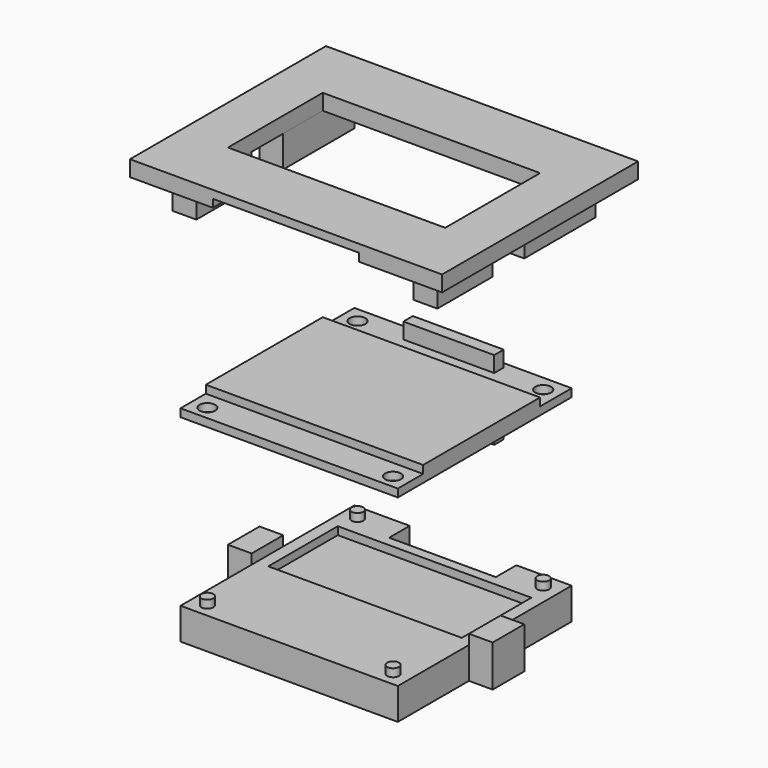
from build123d import *

# Parameters (mm, degrees)
F0_W          = 27.5
F0_H          = 27.5
F0_R          = 1
F1_DEPTH      = 1
F2_W          = 18.5
F2_H          = 1
F3_DEPTH      = 13.75
F3_DEPTH_BACK = 13.75
F4_W          = 11.5
F4_H          = 1.5
F5_DEPTH      = 2
F5_DEPTH_BACK = 8
F6_W          = 23.5
F6_H          = 10
F7_DEPTH      = 0.5
F9_W          = 39.5
F9_H          = 31
F9_W_2        = 27.5000000002
F9_H_2        = 3.5
F10_DEPTH     = 2
F11_W         = 27.5
F11_H         = 3.5
F11_H_2       = 4.5
F11_W_2       = 12.5
F11_H_3       = 2.5
F11_W_3       = 11.5
F11_H_4       = 1.5
F12_DEPTH     = 1
F13_W         = 3
F13_H         = 8.75
F14_DEPTH     = 4
F15_W         = 4.5
F15_H         = 3.5
F16_DEPTH     = 1
F18_W         = 33.5
F18_H         = 27.5
F19_DEPTH     = 4
F20_R         = 0.75
F21_DEPTH     = 1
F22_W         = 3
F22_H         = 5
F23_DEPTH     = 1.25
F24_W         = 3
F24_H         = 11.25
F24_W_2       = 13.5
F24_H_2       = 3.25
F25_DEPTH     = 4
F26_W         = 24.5
F26_H         = 11
F27_DEPTH     = 1


with BuildPart() as f1:
    # F0 (on Top) → F1 (new body)
    with BuildSketch(Plane.XY):
        Rectangle(F0_W, F0_H)
        with Locations((-11.75, -12)):
            Circle(F0_R, mode=Mode.SUBTRACT)
        with Locations((11.75, -12)):
            Circle(F0_R, mode=Mode.SUBTRACT)
        with Locations((-11.75, 11.75)):
            Circle(F0_R, mode=Mode.SUBTRACT)
        with Locations((11.75, 11.75)):
            Circle(F0_R, mode=Mode.SUBTRACT)
    extrude(amount=F1_DEPTH)

    # F2 (on Right) → F3 (join, two sides)
    with BuildSketch(Plane.YZ) as f3_sk:
        with Locations((-0.5, 1.5)):
            Rectangle(F2_W, F2_H)
    extrude(amount=F3_DEPTH)
    extrude(f3_sk.sketch, amount=-F3_DEPTH_BACK)

    # F4 (on face) → F5 (join, two sides)
    with BuildSketch(Plane.XY.offset(1)) as f5_sk:
        with Locations((0, 12.25)):
            Rectangle(F4_W, F4_H)
    extrude(amount=F5_DEPTH)
    extrude(f5_sk.sketch, amount=-F5_DEPTH_BACK)

    # F6 (on face) → F7 (join)
    with BuildSketch(Plane(origin=(0, 0, 0), x_dir=(1, 0, 0), z_dir=(0, 0, -1))):
        with Locations((0, -3.75)):
            Rectangle(F6_W, F6_H)
    extrude(amount=F7_DEPTH)


with BuildPart() as f10:
    # F9 (on offset) → F10 (new body)
    with BuildSketch(Plane.XY.offset(25)):
        with Locations((0, 1.25)):
            Rectangle(F9_W, F9_H)
        Polygon((-13.7499999998, 8.75), (13.7500000002, 8.75), (13.75, -6.25), (13.75, -9.75), (-13.7499999998, -9.75), (-13.75, -6.25), align=None, mode=Mode.SUBTRACT)
        with Locations((1e-10, -8)):
            Rectangle(F9_W_2, F9_H_2)
    extrude(amount=F10_DEPTH)

    # F11 (on face) → F12 (cut)
    with BuildSketch(Plane(origin=(0, 0, 25), x_dir=(1, 0, 0), z_dir=(0, 0, -1))):
        with Locations((0, 8)):
            Rectangle(F11_W, F11_H)
        with Locations((0, 12)):
            Rectangle(F11_W, F11_H_2)
        with Locations((0, -12.25)):
            Rectangle(F11_W_2, F11_H_3)
        with Locations((0, -12.25)):
            Rectangle(F11_W_3, F11_H_4, mode=Mode.SUBTRACT)
        with Locations((0, -12.25)):
            Rectangle(F11_W_3, F11_H_4)
    extrude(amount=-F12_DEPTH, mode=Mode.SUBTRACT)

    # F13 (on face) → F14 (join)
    with BuildSketch(Plane(origin=(0, 0, 25), x_dir=(1, 0, 0), z_dir=(0, 0, -1))):
        with Locations((-15.25, 6.875)):
            Rectangle(F13_W, F13_H)
        Polygon((16.75, -2.5), (13.75, -2.5), (13.75, -8.75), (13.75, -13.75), (16.75, -13.75), align=None)
        Polygon((-13.75, -8.75), (-13.75, -2.5), (-16.75, -2.5), (-16.75, -13.75), (-13.75, -13.75), align=None)
        with Locations((15.25, 6.875)):
            Rectangle(F13_W, F13_H)
    extrude(amount=F14_DEPTH)

    # F15 (on face) → F16 (join, through all)
    with BuildSketch(Plane(origin=(0, 0, 26), x_dir=(1, 0, 0), z_dir=(0, 0, -1))):
        with Locations((-11.5, 12.5)):
            Rectangle(F15_W, F15_H)
        with Locations((11.5, 12.5)):
            Rectangle(F15_W, F15_H)
    extrude(amount=F16_DEPTH)


with BuildPart() as f19:
    # F18 (on offset) → F19 (new body)
    with BuildSketch(Plane.XY.offset(-25)):
        Rectangle(F18_W, F18_H)
    extrude(amount=F19_DEPTH)

    # F20 (on face) → F21 (join)
    with BuildSketch(Plane.XY.offset(-21)):
        with Locations((-11.75, -12)):
            Circle(F20_R)
        with Locations((11.75, -12)):
            Circle(F20_R)
        with Locations((11.75, 11.75)):
            Circle(F20_R)
        with Locations((-11.75, 11.75)):
            Circle(F20_R)
    extrude(amount=F21_DEPTH)

    # F22 (on face) → F23 (join)
    with BuildSketch(Plane.XY.offset(-21)):
        with Locations((-15.25, 0)):
            Rectangle(F22_W, F22_H)
        with Locations((15.25, 0)):
            Rectangle(F22_W, F22_H)
    extrude(amount=F23_DEPTH)

    # F24 (on face) → F25 (cut, through all)
    with BuildSketch(Plane(origin=(0, 0, -25), x_dir=(1, 0, 0), z_dir=(0, 0, -1))):
        with Locations((-15.25, 8.125)):
            Rectangle(F24_W, F24_H)
        with Locations((15.25, -8.125)):
            Rectangle(F24_W, F24_H)
        with Locations((-15.25, -8.125)):
            Rectangle(F24_W, F24_H)
        with Locations((15.25, 8.125)):
            Rectangle(F24_W, F24_H)
        with Locations((0, -12.125)):
            Rectangle(F24_W_2, F24_H_2)
    extrude(amount=-F25_DEPTH, mode=Mode.SUBTRACT)

    # F26 (on face) → F27 (cut)
    with BuildSketch(Plane.XY.offset(-21)):
        with Locations((0, 3.75)):
            Rectangle(F26_W, F26_H)
    extrude(amount=-F27_DEPTH, mode=Mode.SUBTRACT)


solid = Compound([f1.part, f10.part, f19.part])
